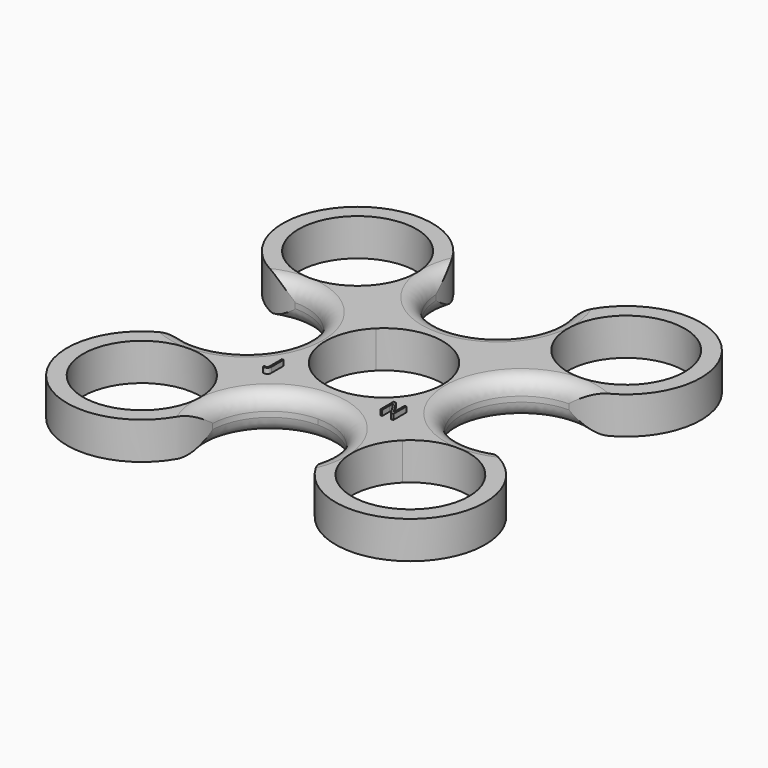
from build123d import *

# Parameters (mm, degrees)
F1_DEPTH       = 7
F2_T2_ANGLE    = 252.4191329241
F2_T4_ANGLE    = 255.9271622092
F2_T6_ANGLE    = 252.4191329241
F2_T8_ANGLE    = 255.9271622092
F2_T10_ANGLE   = 255.9271622092
F2_T12_ANGLE   = 252.4191329241
F2_T14_ANGLE   = 255.9271622092
F2_T16_ANGLE   = 252.4191329241
F3_TEXT_SIZE   = 4.0402364296
F3_TEXT_SIZE_2 = 4.3288274254
F4_DEPTH       = 1


# Not quite as in the source:
# - a fillet or chamfer that OpenCascade refuses, or shapes differently, is made with other operations: its cross-section is extruded or revolved along the edge and cut away or added
# - Text() gives the source's letters only with a copy of the font that has no kerning and outlines rounded to 1/6400 em; it was checked with that copy


with BuildPart() as f1:
    # F0 (on Top) → F1 (new body)
    with BuildSketch(Plane.XY):
        with BuildLine():
            ThreePointArc((0, 15.4721900565), (-7.7910911883, 18.6152071979), (-11.2203173339, 26.2846313417))
            ThreePointArc((-11.2203173339, 26.2846313417), (-35.3267050859, 35.1421211089), (-25.7651731372, 11.3062204081))
            ThreePointArc((-25.7651731372, 11.3062204081), (-14.4795720012, 0), (-25.7651731372, -11.3062204081))
            ThreePointArc((-25.7651731372, -11.3062204081), (-35.3267050859, -35.1421211089), (-11.2203173339, -26.2846313417))
            ThreePointArc((-11.2203173339, -26.2846313417), (-7.7910911883, -18.6152071979), (0, -15.4721900565))
            ThreePointArc((0, -15.4721900565), (7.7910911883, -18.6152071979), (11.2203173339, -26.2846313417))
            ThreePointArc((11.2203173339, -26.2846313417), (35.3267050859, -35.1421211089), (25.7651731372, -11.3062204081))
            ThreePointArc((25.7651731372, -11.3062204081), (14.4795720012, 0), (25.7651731372, 11.3062204081))
            ThreePointArc((25.7651731372, 11.3062204081), (35.3267050859, 35.1421211089), (11.2203173339, 26.2846313417))
            ThreePointArc((11.2203173339, 26.2846313417), (7.7910911883, 18.6152071979), (0, 15.4721900565))
        make_face()
        with BuildLine():
            ThreePointArc((-14.211258501, -25.3510701327), (-35.4320600002, -29.5838441042), (-17.4591726391, -17.5333623019))
            ThreePointArc((-17.4591726391, -17.5333623019), (-15.0555421392, -21.1182961612), (-14.211258501, -25.3510701327))
        make_face(mode=Mode.SUBTRACT)
        with BuildLine():
            ThreePointArc((36.2480030701, -25.3510701327), (21.0219003143, -35.513157304), (17.4791699146, -17.5534445523))
            ThreePointArc((17.4791699146, -17.5534445523), (29.4657018251, -15.1889829614), (36.2480030701, -25.3510701327))
        make_face(mode=Mode.SUBTRACT)
        with BuildLine():
            ThreePointArc((-14.1530308172, 25.3510701327), (-15.0017704255, 21.0959563766), (-17.418086835, 17.4921019109))
            ThreePointArc((-17.418086835, 17.4921019109), (-35.4858317139, 29.6061838888), (-14.1530308172, 25.3510701327))
        make_face(mode=Mode.SUBTRACT)
        with BuildLine():
            ThreePointArc((-7.7878811866, -7.8209744087), (-11.0371524443, 0), (-7.7878811866, 7.8209744087))
            ThreePointArc((-7.7878811866, 7.8209744087), (0, 11.0371524443), (7.7878811866, 7.8209744087))
            ThreePointArc((7.7878811866, 7.8209744087), (10.1925160278, 4.2345426084), (11.0371524443, 0))
            ThreePointArc((11.0371524443, 0), (10.1925160278, -4.2345426084), (7.7878811866, -7.8209744087))
            ThreePointArc((7.7878811866, -7.8209744087), (0, -11.0371524443), (-7.7878811866, -7.8209744087))
        make_face(mode=Mode.SUBTRACT)
        with BuildLine():
            ThreePointArc((36.2449954382, 25.3510701327), (29.4645479092, 15.1917604292), (17.4812921178, 17.5555757734))
            ThreePointArc((17.4812921178, 17.5555757734), (21.0230542302, 35.5103798361), (36.2449954382, 25.3510701327))
        make_face(mode=Mode.SUBTRACT)
    extrude(amount=F1_DEPTH)

    # F2: fillet of radius 3 on 8 edges, made by hand

    # F2_s1 → F2_t2 (revolve, cut)
    with BuildSketch(Plane(origin=(12.7265382439, 17.3825190325, 0), x_dir=(0, 0, 1), z_dir=(0.5907403945, 0.8068616897, 0))):
        with BuildLine():
            ThreePointArc((7, -30.0008974416), (6.1213203436, -27.8795770981), (4, -27.0008974416))
            Line((4, -27.0008974416), (7, -27.0008974416))
            Line((7, -27.0008974416), (7, -30.0008974416))
        make_face()
    revolve(axis=Axis((0, 26.700200513, 7), (0, 0, 1)), revolution_arc=F2_T2_ANGLE, mode=Mode.SUBTRACT)

    # F2_s3 → F2_t4 (revolve, cut)
    with BuildSketch(Plane(origin=(-16.0278826321, -12.5059559629, 0), x_dir=(0, 0, 1), z_dir=(-0.7884019271, -0.615160468, 0))):
        with BuildLine():
            ThreePointArc((7, 30.1686509578), (6.1213203436, 28.0473306142), (4, 27.1686509578))
            Line((4, 27.1686509578), (7, 27.1686509578))
            Line((7, 27.1686509578), (7, 30.1686509578))
        make_face()
    revolve(axis=Axis((-25.7858112454, 0, 7), (0, 0, -1)), revolution_arc=F2_T4_ANGLE, mode=Mode.SUBTRACT)

    # F2_s5 → F2_t6 (revolve, cut)
    with BuildSketch(Plane(origin=(-12.7265382439, -17.3825190325, 0), x_dir=(0, 0, 1), z_dir=(-0.5907403945, -0.8068616897, 0))):
        with BuildLine():
            ThreePointArc((7, -30.0008974416), (6.1213203436, -27.8795770981), (4, -27.0008974416))
            Line((4, -27.0008974416), (7, -27.0008974416))
            Line((7, -27.0008974416), (7, -30.0008974416))
        make_face()
    revolve(axis=Axis((0, -26.700200513, 7), (0, 0, 1)), revolution_arc=F2_T6_ANGLE, mode=Mode.SUBTRACT)

    # F2_s7 → F2_t8 (revolve, cut)
    with BuildSketch(Plane(origin=(16.0278826321, 12.5059559629, 0), x_dir=(0, 0, 1), z_dir=(0.7884019271, 0.615160468, 0))):
        with BuildLine():
            ThreePointArc((0, 30.1686509578), (0.8786796564, 28.0473306142), (3, 27.1686509578))
            Line((3, 27.1686509578), (0, 27.1686509578))
            Line((0, 27.1686509578), (0, 30.1686509578))
        make_face()
    revolve(axis=Axis((25.7858112454, 0, 0), (0, 0, -1)), revolution_arc=F2_T8_ANGLE, mode=Mode.SUBTRACT)

    # F2_s9 → F2_t10 (revolve, cut)
    with BuildSketch(Plane(origin=(16.0278826321, 12.5059559629, 0), x_dir=(0, 0, 1), z_dir=(0.7884019271, 0.615160468, 0))):
        with BuildLine():
            ThreePointArc((7, 30.1686509578), (6.1213203436, 28.0473306142), (4, 27.1686509578))
            Line((4, 27.1686509578), (7, 27.1686509578))
            Line((7, 27.1686509578), (7, 30.1686509578))
        make_face()
    revolve(axis=Axis((25.7858112454, 0, 7), (0, 0, -1)), revolution_arc=F2_T10_ANGLE, mode=Mode.SUBTRACT)

    # F2_s11 → F2_t12 (revolve, cut)
    with BuildSketch(Plane(origin=(12.7265382439, -17.3825190325, 0), x_dir=(0, 0, 1), z_dir=(0.5907403945, -0.8068616897, 0))):
        with BuildLine():
            ThreePointArc((3, 27.0008974416), (0.8786796564, 27.8795770981), (0, 30.0008974416))
            Line((0, 30.0008974416), (0, 27.0008974416))
            Line((0, 27.0008974416), (3, 27.0008974416))
        make_face()
    revolve(axis=Axis((0, -26.700200513, 0), (0, 0, -1)), revolution_arc=F2_T12_ANGLE, mode=Mode.SUBTRACT)

    # F2_s13 → F2_t14 (revolve, cut)
    with BuildSketch(Plane(origin=(-16.0278826321, -12.5059559629, 0), x_dir=(0, 0, 1), z_dir=(-0.7884019271, -0.615160468, 0))):
        with BuildLine():
            ThreePointArc((3, 27.1686509578), (0.8786796564, 28.0473306142), (0, 30.1686509578))
            Line((0, 30.1686509578), (0, 27.1686509578))
            Line((0, 27.1686509578), (3, 27.1686509578))
        make_face()
    revolve(axis=Axis((-25.7858112454, 0, 0), (0, 0, -1)), revolution_arc=F2_T14_ANGLE, mode=Mode.SUBTRACT)

    # F2_s15 → F2_t16 (revolve, cut)
    with BuildSketch(Plane(origin=(-12.7265382439, 17.3825190325, 0), x_dir=(0, 0, 1), z_dir=(-0.5907403945, 0.8068616897, 0))):
        with BuildLine():
            ThreePointArc((0, 30.0008974416), (0.8786796564, 27.8795770981), (3, 27.0008974416))
            Line((3, 27.0008974416), (0, 27.0008974416))
            Line((0, 27.0008974416), (0, 30.0008974416))
        make_face()
    revolve(axis=Axis((0, 26.700200513, 0), (0, 0, -1)), revolution_arc=F2_T16_ANGLE, mode=Mode.SUBTRACT)

    # F3 (on face) → F4 (join)
    with BuildSketch(Plane.XY.offset(7)):
        with Locations((-11.6094239056, -12.824931182)):
            Text('J', F3_TEXT_SIZE, font='Open Sans', text_align=(TextAlign.LEFT, TextAlign.BOTTOM))
        with Locations((9.5845097676, -13.3443912491)):
            Text('N', F3_TEXT_SIZE_2, font='Open Sans', text_align=(TextAlign.LEFT, TextAlign.BOTTOM))
    extrude(amount=F4_DEPTH)


solid = f1.part
